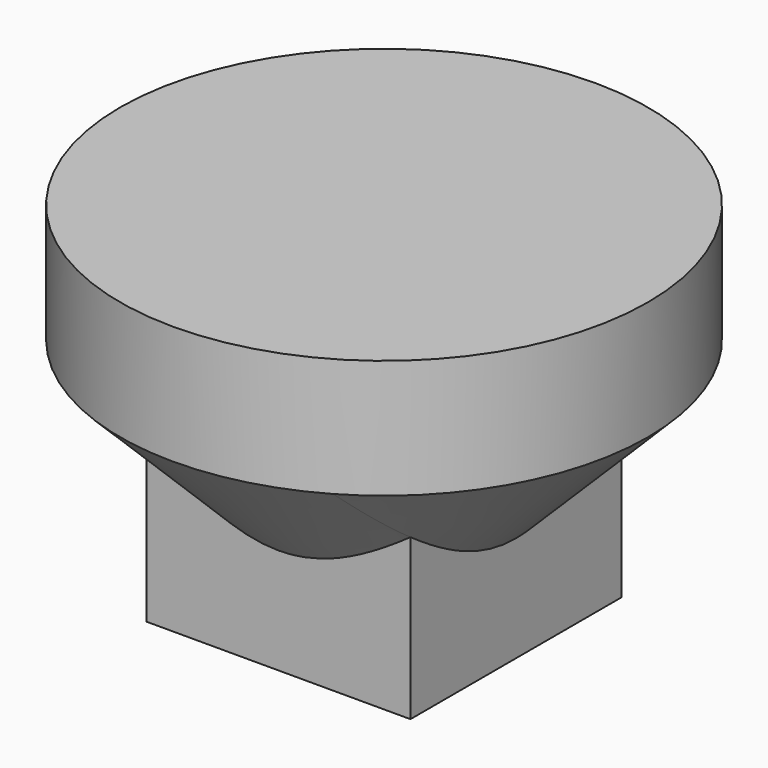
from build123d import *

# Parameters (mm, degrees)
F0_W     = 41
F0_H     = 41
F0_W_2   = 10
F0_H_2   = 10
F1_DEPTH = 10
F2_DEPTH = 25
F3_R     = 10
F4_DEPTH = 8
F6_DEPTH = 25
F7_DEPTH = 1.5
F8_DEPTH = 10
F9_DEPTH = 3


# Not quite as in the source:
# - a fillet or chamfer that OpenCascade refuses, or shapes differently, is made with other operations: its cross-section is extruded or revolved along the edge and cut away or added


with BuildPart() as f1:
    # F0 (on Top) → F1 (new body)
    with BuildSketch(Plane.XY):
        Rectangle(F0_W, F0_H)
        Rectangle(F0_W_2, F0_H_2, mode=Mode.SUBTRACT)
        Rectangle(F0_W_2, F0_H_2)
    extrude(amount=F1_DEPTH)

    # F0 (on Top) → F2 (join)
    with BuildSketch(Plane.XY):
        Rectangle(F0_W_2, F0_H_2)
    extrude(amount=F2_DEPTH)

    # F3 (on face) → F4 (join)
    with BuildSketch(Plane.XY.offset(25)):
        Circle(F3_R)
    extrude(amount=-F4_DEPTH)

    # F5 (on face) → F6 (cut)
    with BuildSketch(Plane(origin=(0, 0, 0), x_dir=(1, 0, 0), z_dir=(0, 0, -1))):
        with BuildLine():
            Line((0, 20.5), (0, 16.625))
            ThreePointArc((0, 16.625), (14.2014511666, 13.1849661001), (20.5, 0))
            Line((20.5, 0), (20.5, 20.5))
            Line((20.5, 20.5), (0, 20.5))
        make_face()
        with BuildLine():
            Line((20.5, -20.5), (20.5, 0))
            Line((20.5, 0), (16.625, 0))
            ThreePointArc((16.625, 0), (13.15340166, -14.1758531755), (0, -20.5))
            Line((0, -20.5), (20.5, -20.5))
        make_face()
        with BuildLine():
            ThreePointArc((0, -16.625), (-14.1919455674, -13.1732449101), (-20.5, 0))
            Line((-20.5, 0), (-20.5, -20.5))
            Line((-20.5, -20.5), (0, -20.5))
            Line((0, -20.5), (0, -16.625))
        make_face()
        with BuildLine():
            ThreePointArc((-16.625, 0), (-13.1636820987, 14.1841903605), (0, 20.5))
            Line((0, 20.5), (-20.5, 20.5))
            Line((-20.5, 20.5), (-20.5, 0))
            Line((-20.5, 0), (-16.625, 0))
        make_face()
    extrude(amount=-F6_DEPTH, mode=Mode.SUBTRACT)

    # F7 (cut): a face of the model
    f7_faces = [f1.faces().sort_by_distance(p)[0] for p in [
        (0, 0, 25),
    ]]
    extrude(f7_faces, amount=-F7_DEPTH, mode=Mode.SUBTRACT)

    # F8 (cut): a face of the model
    f8_faces = [f1.faces().sort_by_distance(p)[0] for p in [
        (0.0007164835, -0.0062799282, 0),
    ]]
    extrude(f8_faces, amount=-F8_DEPTH, mode=Mode.SUBTRACT)

    # F9 (add): a face of the model
    f9_faces = [f1.faces().sort_by_distance(p)[0] for p in [
        (-9.7171572875, 0, 17),
    ]]
    extrude(f9_faces, amount=F9_DEPTH)

    # F10: chamfer of 5 on 1 edges, made by hand


with BuildPart() as f10_tool2:
    # F10_s3 → F10_t4 (revolve)
    with BuildSketch(Plane.XZ):
        Polygon((5, 14), (10, 19), (10, 14), align=None)
    revolve(axis=Axis((0, 0, 14), (0, 0, 1)))

    split(bisect_by=Plane.YZ.offset(5), keep=Keep.TOP)


with BuildPart() as f1_1:
    add(f1.part)

    # F10_t1: cut F10_tool2
    add(f10_tool2.part, mode=Mode.SUBTRACT)


with BuildPart() as f10_tool7:
    # F10_s8 → F10_t9 (revolve)
    with BuildSketch(Plane.XZ):
        Polygon((5, 14), (10, 19), (10, 14), align=None)
    revolve(axis=Axis((0, 0, 14), (0, 0, 1)))

    split(bisect_by=Plane.XZ.offset(-5), keep=Keep.BOTTOM)


with BuildPart() as f1_2:
    add(f1_1.part)

    # F10_t6: cut F10_tool7
    add(f10_tool7.part, mode=Mode.SUBTRACT)


with BuildPart() as f10_tool12:
    # F10_s13 → F10_t14 (revolve)
    with BuildSketch(Plane.XZ):
        Polygon((5, 14), (10, 19), (10, 14), align=None)
    revolve(axis=Axis((0, 0, 14), (0, 0, 1)))

    split(bisect_by=Plane.YZ.offset(-5), keep=Keep.BOTTOM)


with BuildPart() as f1_3:
    add(f1_2.part)

    # F10_t11: cut F10_tool12
    add(f10_tool12.part, mode=Mode.SUBTRACT)


with BuildPart() as f10_tool17:
    # F10_s18 → F10_t19 (revolve)
    with BuildSketch(Plane.XZ):
        Polygon((5, 14), (10, 19), (10, 14), align=None)
    revolve(axis=Axis((0, 0, 14), (0, 0, 1)))

    split(bisect_by=Plane.XZ.offset(5), keep=Keep.TOP)


with BuildPart() as f1_4:
    add(f1_3.part)

    # F10_t16: cut F10_tool17
    add(f10_tool17.part, mode=Mode.SUBTRACT)


solid = f1_4.part
